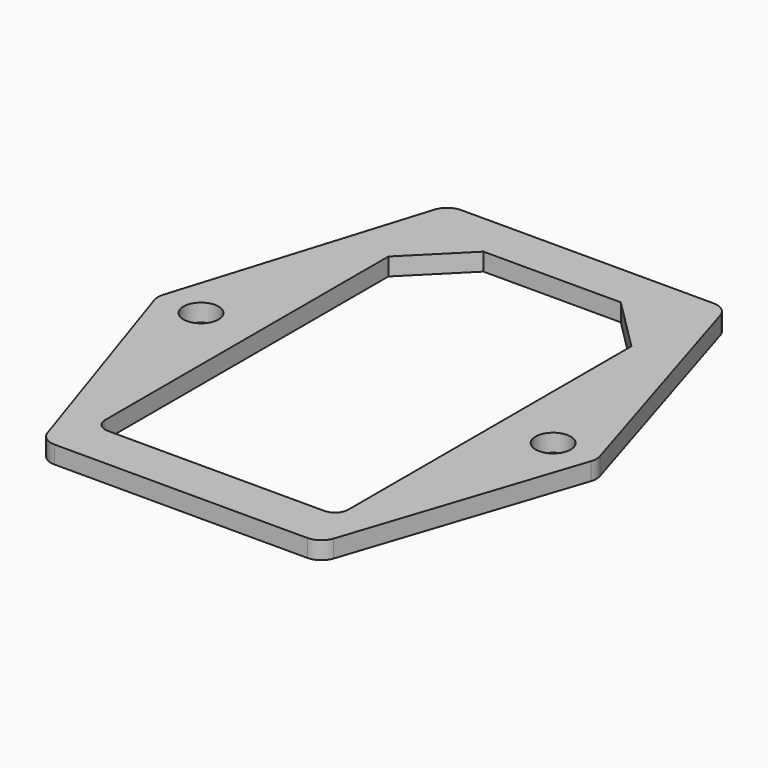
from build123d import *

# Parameters (mm, degrees)
F0_W     = 31.6
F0_H     = 57.7
F0_R     = 2
F1_DEPTH = 2
F2_R     = 1.5
F3_R     = 2


# Not quite as in the source:
# - a feature names something its author has since deleted; it is built from what else it names


with BuildPart() as f1:
    # F0 (on Top) → F1 (new body)
    with BuildSketch(Plane.XY):
        Rectangle(F0_W, F0_H)
        Polygon((7.8, 23.85), (13.8, 23.85), (13.8, 17.85), (13.8, -23.85), (-13.8, -23.85), (-13.8, 17.85), (-13.8, 23.85), (-7.8, 23.85), align=None, mode=Mode.SUBTRACT)
        Polygon((-15.8, -28.85), (-15.8, 28.85), (-25, -1), align=None)
        with Locations((-20, -1)):
            Circle(F0_R, mode=Mode.SUBTRACT)
        Polygon((25, -1), (15.8, 28.85), (15.8, -28.85), align=None)
        with Locations((20, -1)):
            Circle(F0_R, mode=Mode.SUBTRACT)
        Polygon((-13.8, 17.85), (-7.8, 23.85), (-13.8, 23.85), align=None)
        Polygon((13.8, 17.85), (13.8, 23.85), (7.8, 23.85), align=None)
    extrude(amount=F1_DEPTH)

    # F2
    f2_edges = [f1.edges().sort_by_distance(p)[0] for p in [
        (13.8, -23.85, 1),
        (-13.8, -23.85, 1),
    ]]
    fillet(f2_edges, radius=F2_R)

    # F3
    f3_edges = [f1.edges().sort_by_distance(p)[0] for p in [
        (15.8, -28.85, 1),
        (-15.8, -28.85, 1),
        (25, -1, 1),
        (15.8, 28.85, 1),
        (-15.8, 28.85, 1),
        (-25, -1, 1),
    ]]
    fillet(f3_edges, radius=F3_R)


solid = f1.part
